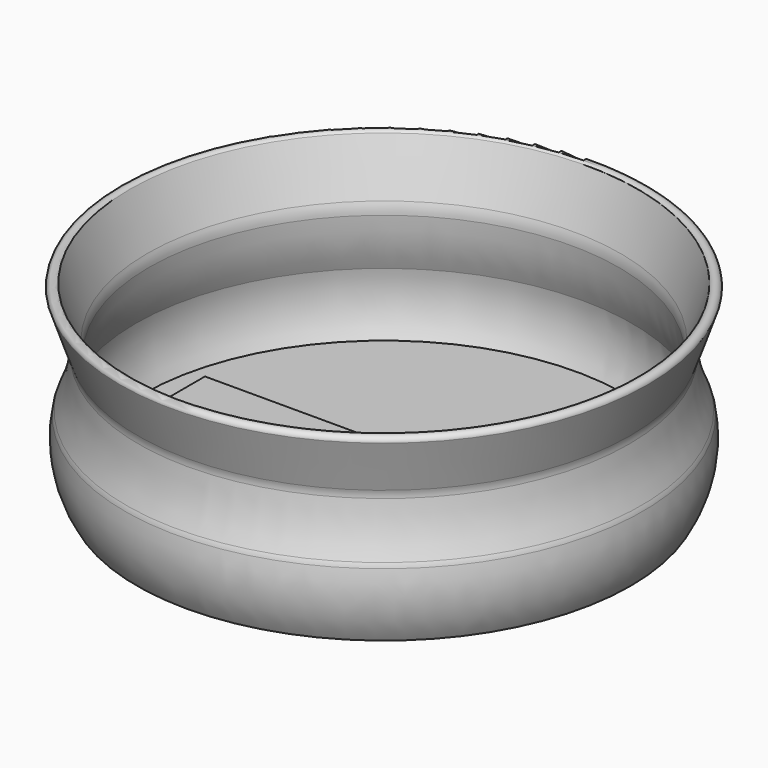
from build123d import *

# Parameters (mm, degrees)
F2_TEXT_SIZE = 35.1982475776
F3_DEPTH     = 2.54


# Not quite as in the source:
# - Text() gives the source's letters only with a copy of the font that has no kerning and outlines rounded to 1/6400 em; it was checked with that copy


with BuildPart() as f1:
    # F0 (on Front) → F1 (revolve)
    with BuildSketch(Plane.XZ):
        with BuildLine():
            Line((-76.2, 0), (0, 0))
            Line((0, 0), (0, 3.175))
            Line((0, 3.175), (-74.3391473358, 3.175))
            ThreePointArc((-74.3391473358, 3.175), (-77.1979952453, 12.5981888377), (-76.5029277219, 22.420936945))
            ThreePointArc((-76.5029277219, 22.420936945), (-76.5457364486, 22.0068029341), (-76.6220522644, 21.5975164057))
            ThreePointArc((-76.6220522644, 21.5975164057), (-73.7880668932, 29.6916530957), (-72.5352875092, 38.1755829432))
            ThreePointArc((-72.5352875092, 38.1755829432), (-72.6179989804, 40.0103805933), (-73.0513200149, 41.7951933245))
            Line((-73.0513200149, 41.7951933245), (-78.4928197253, 57.4395080332))
            ThreePointArc((-78.4928197253, 57.4395080332), (-80.351259836, 57.9502546487), (-81.4915971178, 56.3964552299))
            Line((-81.4915971178, 56.3964552299), (-76.0500974074, 40.7521405212))
            ThreePointArc((-76.0500974074, 40.7521405212), (-75.7612167177, 39.562265367), (-75.7060757369, 38.3390669336))
            ThreePointArc((-75.7060757369, 38.3390669336), (-76.8707795801, 30.4515922316), (-79.5055241293, 22.9265066256))
            ThreePointArc((-79.5055241293, 22.9265066256), (-79.7791007004, 22.2267433585), (-79.9681103213, 21.4995651593))
            ThreePointArc((-79.9681103213, 21.4995651593), (-80.0879917907, 10.3985636483), (-76.2, 0))
        make_face()
    revolve(axis=Axis((0, 0, 1.5875), (0, 0, 1)))

    # F2 (on face) → F3 (join)
    with BuildSketch(Plane.XY.offset(3.175)):
        Polygon((65.3559961075, 12.6713691279), (-65.3559961075, 12.6713691279), (-65.3559961075, -12.6713691279), (-62.1936535517, -12.6713691279), (-62.1936535517, 12.4568798068), (-47.7898706758, 12.4568798068), (-47.7898706758, 8.0900972167), (-56.9524144984, 8.0900972167), (-56.9524144984, 1.6114197719), (-48.4278389132, 1.6114197719), (-48.4278389132, -2.7388636396), (-56.9524144984, -2.7388636396), (-56.9524144984, -12.6713691279), (-42.8731154673, -12.6713691279), (-42.8731154673, 12.4568798068), (-37.5438807951, 12.4568798068), (-37.5438807951, -12.6713691279), (-31.2191956835, -12.6713691279), (-31.2191956835, 12.4568798068), (-25.8899610112, 12.4568798068), (-25.8899610112, -8.2715881807), (-15.6989683922, -8.2715881807), (-15.6989683922, -12.6713691279), (-11.3321858021, -12.6713691279), (-11.3321858021, 12.4568798068), (-6.0029511298, 12.4568798068), (-6.0029511298, -8.2715881807), (4.1880414891, -8.2715881807), (4.1880414891, -12.6713691279), (17.7008687232, -12.6713691279), (17.7008687232, 12.4568798068), (24.9550075599, 12.4568798068), (30.9002115648, -6.7591634801), (31.0047063623, -6.7591634801), (37.3128922953, 12.4568798068), (44.5615314058, 12.4568798068), (44.5615314058, -12.6713691279), (50.8862165174, -12.6713691279), (50.8862165174, 12.4568798068), (65.3559961075, 12.4568798068), align=None)
        Polygon((65.3559961075, -8.2715881807), (65.3559961075, 8.0900972167), (56.2154511897, 8.0900972167), (56.2154511897, 2.5738718541), (64.7235275964, 2.5738718541), (64.7235275964, -1.792910736), (56.2154511897, -1.792910736), (56.2154511897, -8.2715881807), align=None)
        with BuildLine():
            Line((33.2210960144, -12.6713691279), (39.5952786617, -12.6713691279))
            Line((39.5952786617, -12.6713691279), (39.5952786617, -0.7754613919))
            add(Edge.make_bspline(
                [(39.5952786617, -0.7754613919), (39.5952786617, 0.0659967142), (39.6227772926, 1.165941951)],
                knots=[0, 0, 0, 1, 1, 1], degree=2))
            add(Edge.make_bspline(
                [(39.6227772926, 1.165941951), (39.6502759235, 2.2658871878), (39.8537657923, 7.0066511584)],
                knots=[0, 0, 0, 1, 1, 1], degree=2))
            Line((39.8537657923, 7.0066511584), (39.6997734592, 7.0066511584))
            Line((39.6997734592, 7.0066511584), (33.2210960144, -12.6713691279))
        make_face()
        with BuildLine():
            Line((22.4636315985, -12.6713691279), (28.337339163, -12.6713691279))
            Line((28.337339163, -12.6713691279), (22.2876403606, 7.0396495155))
            Line((22.2876403606, 7.0396495155), (22.1336480275, 7.0396495155))
            add(Edge.make_bspline(
                [(22.1336480275, 7.0396495155), (22.4636315985, 1.0284487964), (22.4636315985, -0.9844509869)],
                knots=[0, 0, 0, 1, 1, 1], degree=2))
            Line((22.4636315985, -0.9844509869), (22.4636315985, -12.6713691279))
        make_face()
        with Locations((-65.3559961075, -12.6713691279)):
            Text('FILL ME', F2_TEXT_SIZE, font='Open Sans', font_style=FontStyle.BOLD, text_align=(TextAlign.LEFT, TextAlign.BOTTOM))
    extrude(amount=F3_DEPTH)


solid = f1.part
